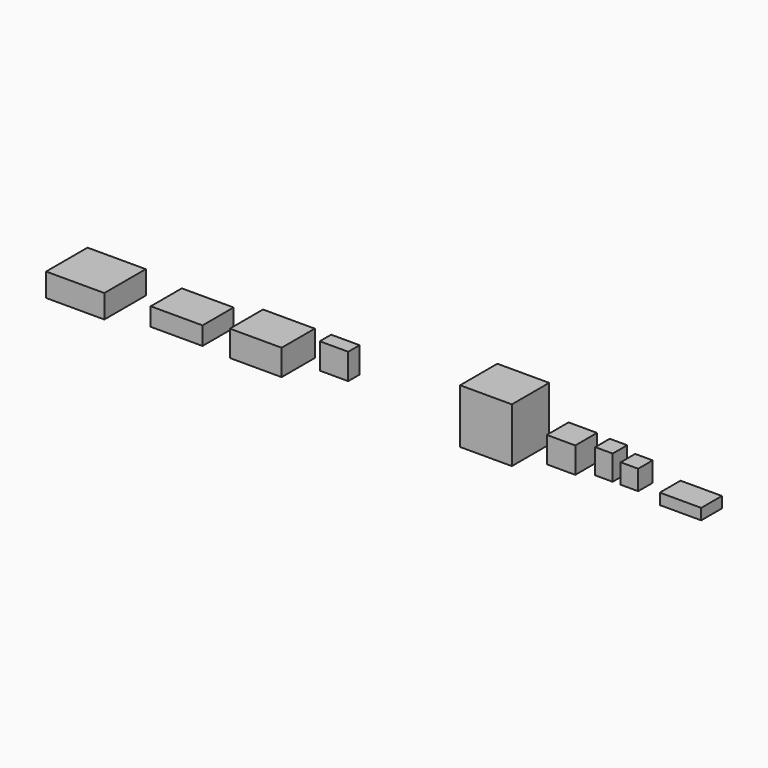
from build123d import *

# Parameters (mm, degrees)
F0_W          = 1143
F0_H          = 1016
F1_DEPTH      = 457.2
F0_W_2        = 1016
F0_H_2        = 762
F2_DEPTH      = 355.6
F0_H_3        = 812.8
F3_DEPTH      = 508
F0_W_3        = 558.8
F0_H_4        = 279.4
F4_DEPTH      = 508
F0_H_5        = 914.4
F6_DEPTH      = 1066.8
F0_H_6        = 533.4
F7_DEPTH      = 508
F0_W_4        = 342.9
F0_H_7        = 355.6
F8_DEPTH      = 487.68
F9_DEPTH      = 388.62
F0_W_5        = 812.8
F0_H_8        = 508
F10_DEPTH     = 215.9
F11_TEXT_SIZE = 137.8517287473
F12_DEPTH     = 25.4


# Not quite as in the source:
# - a feature of the source that left no trace in its solid (it failed there, or was rolled back) is left out
# - Text() gives the source's letters only with a copy of the font that has no kerning and outlines rounded to 1/6400 em; it was checked with that copy


with BuildPart() as f1:
    # F0 (on Top) → F1 (new body)
    with BuildSketch(Plane.XY):
        with Locations((-6231.5076073408, -5632.3205070496)):
            Rectangle(F0_W, F0_H)
    extrude(amount=F1_DEPTH)


with BuildPart() as f2:
    # F0 (on Top) → F2 (new body)
    with BuildSketch(Plane.XY):
        with Locations((-4445.1691074371, -5505.3205070496)):
            Rectangle(F0_W_2, F0_H_2)
    extrude(amount=F2_DEPTH)


with BuildPart() as f3:
    # F0 (on Top) → F3 (new body)
    with BuildSketch(Plane.XY):
        with Locations((-2852.6197834015, -5530.7205070496)):
            Rectangle(F0_W_2, F0_H_3)
    extrude(amount=F3_DEPTH)


with BuildPart() as f4:
    # F0 (on Top) → F4 (new body)
    with BuildSketch(Plane.XY):
        with Locations((-1743.884137249, -5264.0205070496)):
            Rectangle(F0_W_3, F0_H_4)
    extrude(amount=F4_DEPTH)


with BuildPart() as f6:
    # F0 (on Top) → F6 (new body)
    with BuildSketch(Plane.XY):
        with Locations((1745.7537488937, -5581.5205070496)):
            Rectangle(F0_W_2, F0_H_5)
    extrude(amount=F6_DEPTH)


with BuildPart() as f7:
    # F0 (on Top) → F7 (new body)
    with BuildSketch(Plane.XY):
        with Locations((2913.6732906342, -5391.0205070496)):
            Rectangle(F0_W_3, F0_H_6)
    extrude(amount=F7_DEPTH)

    # F11 (on face) → F12 (join)
    with BuildSketch(Plane(origin=(0, -5124.3205070496, 0), x_dir=(-1, 0, 0), z_dir=(0, 1, 0))):
        with Locations((-3138.8330459595, 61.0310584307)):
            Text('FRONT', F11_TEXT_SIZE, font='Open Sans', text_align=(TextAlign.LEFT, TextAlign.BOTTOM))
    extrude(amount=F12_DEPTH)


with BuildPart() as f8:
    # F0 (on Top) → F8 (new body)
    with BuildSketch(Plane.XY):
        with Locations((3613.0481769562, -5302.1205070496)):
            Rectangle(F0_W_4, F0_H_7)
    extrude(amount=F8_DEPTH)


with BuildPart() as f9:
    # F0 (on Top) → F9 (new body)
    with BuildSketch(Plane.XY):
        with Locations((4113.0763103485, -5302.1205070496)):
            Rectangle(F0_W_4, F0_H_7)
    extrude(amount=F9_DEPTH)


with BuildPart() as f10:
    # F0 (on Top) → F10 (new body)
    with BuildSketch(Plane.XY):
        with Locations((5236.7089141846, -5378.3205070496)):
            Rectangle(F0_W_5, F0_H_8)
    extrude(amount=F10_DEPTH)


solid = Compound([f1.part, f2.part, f3.part, f4.part, f6.part, f7.part, f8.part, f9.part, f10.part])
